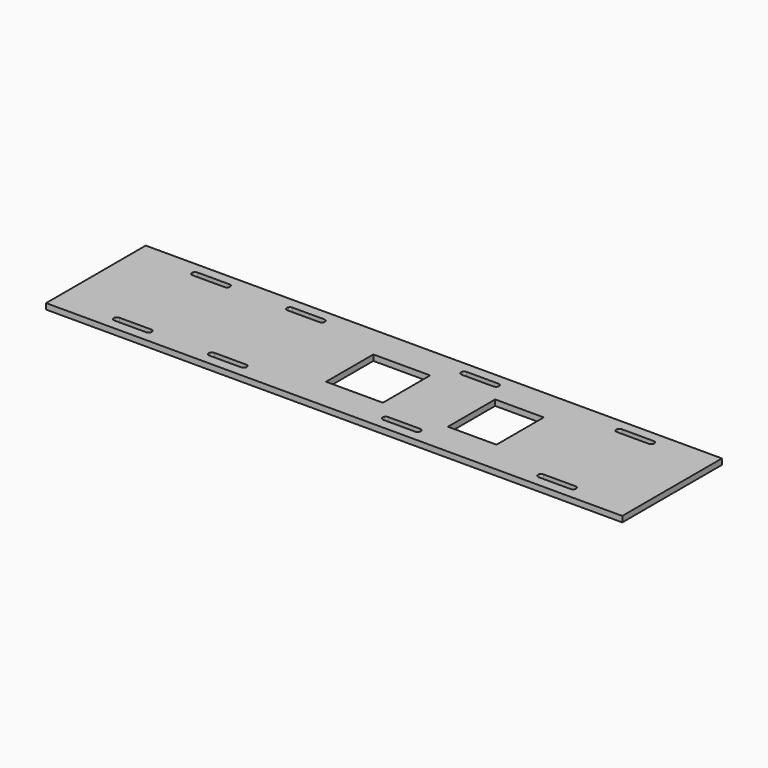
from build123d import *

# Parameters (mm, degrees)
F0_W     = 240.88725
F0_H     = 52.080583
F0_W_2   = 23.749
F0_H_2   = 24.712083
F0_W_3   = 20.32
F1_DEPTH = 2.4


# Not quite as in the source:
# - ends of sketch curves that miss each other by under 0.0002 mm in the source are joined


with BuildPart() as f1:
    # F0 (on Top) → F1 (new body)
    with BuildSketch(Plane.XY):
        with Locations((0, 5e-07)):
            Rectangle(F0_W, F0_H)
        with BuildLine():
            add(Edge.make_bspline(
                [(-95.3406640139, -19.1717048442), (-95.7930787698, -19.173702026), (-96.2109496029, -19.415645799), (-96.438113, -19.80762)],
                knots=[0.0087343308, 0.0087343308, 0.0087343308, 0.0087343308, 1, 1, 1, 1], degree=3))
            Line((-95.3406640139, -19.1717048442), (-95.328697, -19.171708))
            Line((-95.328697, -19.171708), (-82.016247, -19.171708))
            add(Edge.make_bspline(
                [(-80.906831, -19.807617), (-81.135996, -19.412192), (-81.559244, -19.16956), (-82.016247, -19.171708)],
                knots=[0, 0, 0, 0, 1, 1, 1, 1], degree=3))
            add(Edge.make_bspline(
                [(-80.906831, -21.086383), (-80.677667, -20.690913), (-80.677667, -20.203086), (-80.906831, -19.807617)],
                knots=[0, 0, 0, 0, 1, 1, 1, 1], degree=3))
            add(Edge.make_bspline(
                [(-82.0155410145, -21.7222942934), (-81.5588081414, -21.7242989555), (-81.1358779896, -21.4816033731), (-80.906831, -21.086383)],
                knots=[0.0005149583, 0.0005149583, 0.0005149583, 0.0005149583, 1, 1, 1, 1], degree=3))
            add(Edge.make_bspline(
                [(-82.016247, -21.722291), (-82.0160116625, -21.7222921628), (-82.015776334, -21.7222932606), (-82.0155410145, -21.7222942934)],
                knots=[0, 0, 0, 0, 0.0005149583, 0.0005149583, 0.0005149583, 0.0005149583], degree=3))
            Line((-82.016247, -21.722291), (-95.328697, -21.722291))
            add(Edge.make_bspline(
                [(-95.339958014, -21.7222944098), (-95.336206682, -21.7223097734), (-95.3324529811, -21.7223086538), (-95.328697, -21.722291)],
                knots=[0.991781277, 0.991781277, 0.991781277, 0.991781277, 1, 1, 1, 1], degree=3))
            add(Edge.make_bspline(
                [(-96.438113, -21.086383), (-96.2108314436, -21.4785571197), (-95.7926440063, -21.7204404289), (-95.339958014, -21.7222944098)],
                knots=[0, 0, 0, 0, 0.991781277, 0.991781277, 0.991781277, 0.991781277], degree=3))
            add(Edge.make_bspline(
                [(-96.438113, -19.80762), (-96.667277, -20.203086), (-96.667277, -20.690913), (-96.438113, -21.086383)],
                knots=[0, 0, 0, 0, 1, 1, 1, 1], degree=3))
        make_face(mode=Mode.SUBTRACT)
        with BuildLine():
            add(Edge.make_bspline(
                [(-55.6425800139, -19.1717048399), (-56.0949941873, -19.1737016787), (-56.5128664399, -19.4156455176), (-56.74003, -19.80762)],
                knots=[0.0087336193, 0.0087336193, 0.0087336193, 0.0087336193, 1, 1, 1, 1], degree=3))
            Line((-55.6425800139, -19.1717048399), (-55.630614, -19.171708))
            Line((-55.630614, -19.171708), (-42.30758, -19.171708))
            add(Edge.make_bspline(
                [(-41.198165, -19.807617), (-41.427329, -19.412192), (-41.850578, -19.16956), (-42.30758, -19.171708)],
                knots=[0, 0, 0, 0, 1, 1, 1, 1], degree=3))
            add(Edge.make_bspline(
                [(-41.198165, -21.086383), (-40.969, -20.690913), (-40.969, -20.203086), (-41.198165, -19.807617)],
                knots=[0, 0, 0, 0, 1, 1, 1, 1], degree=3))
            add(Edge.make_bspline(
                [(-42.3068750144, -21.722294289), (-41.8501427567, -21.7242993092), (-41.427211157, -21.4816036611), (-41.198165, -21.086383)],
                knots=[0.00051423, 0.00051423, 0.00051423, 0.00051423, 1, 1, 1, 1], degree=3))
            add(Edge.make_bspline(
                [(-42.30758, -21.722291), (-42.3073449959, -21.7222921611), (-42.3071100007, -21.7222932575), (-42.3068750144, -21.722294289)],
                knots=[0, 0, 0, 0, 0.00051423, 0.00051423, 0.00051423, 0.00051423], degree=3))
            Line((-42.30758, -21.722291), (-55.630614, -21.722291))
            add(Edge.make_bspline(
                [(-55.641875014, -21.7222944097), (-55.6381236819, -21.7223097734), (-55.6343699809, -21.7223086539), (-55.630614, -21.722291)],
                knots=[0.9917812593, 0.9917812593, 0.9917812593, 0.9917812593, 1, 1, 1, 1], degree=3))
            add(Edge.make_bspline(
                [(-56.74003, -21.086383), (-56.5127484477, -21.4785571127), (-56.0945600376, -21.7204404203), (-55.641875014, -21.7222944097)],
                knots=[0, 0, 0, 0, 0.9917812593, 0.9917812593, 0.9917812593, 0.9917812593], degree=3))
            add(Edge.make_bspline(
                [(-56.74003, -19.80762), (-56.969194, -20.203086), (-56.969194, -20.690913), (-56.74003, -21.086383)],
                knots=[0, 0, 0, 0, 1, 1, 1, 1], degree=3))
        make_face(mode=Mode.SUBTRACT)
        with BuildLine():
            add(Edge.make_bspline(
                [(17.0966689861, -19.1717048443), (16.644255197, -19.1737020352), (16.2263833928, -19.4156458064), (15.99922, -19.80762)],
                knots=[0.0087343496, 0.0087343496, 0.0087343496, 0.0087343496, 1, 1, 1, 1], degree=3))
            Line((17.0966689861, -19.1717048443), (17.108636, -19.171708))
            Line((17.108636, -19.171708), (30.421086, -19.171708))
            add(Edge.make_bspline(
                [(31.530502, -19.807617), (31.301338, -19.412192), (30.878089, -19.16956), (30.421086, -19.171708)],
                knots=[0, 0, 0, 0, 1, 1, 1, 1], degree=3))
            add(Edge.make_bspline(
                [(31.530502, -21.086383), (31.759666, -20.690913), (31.759666, -20.203086), (31.530502, -19.807617)],
                knots=[0, 0, 0, 0, 1, 1, 1, 1], degree=3))
            add(Edge.make_bspline(
                [(30.4217919855, -21.7222942934), (30.8785248597, -21.7242989555), (31.3014560099, -21.4816033731), (31.530502, -21.086383)],
                knots=[0.0005149583, 0.0005149583, 0.0005149583, 0.0005149583, 1, 1, 1, 1], degree=3))
            add(Edge.make_bspline(
                [(30.421086, -21.722291), (30.4213213375, -21.7222921628), (30.421556666, -21.7222932606), (30.4217919855, -21.7222942934)],
                knots=[0, 0, 0, 0, 0.0005149583, 0.0005149583, 0.0005149583, 0.0005149583], degree=3))
            Line((30.421086, -21.722291), (17.108636, -21.722291))
            add(Edge.make_bspline(
                [(17.097374986, -21.7222944097), (17.1011263181, -21.7223097734), (17.1048800191, -21.7223086539), (17.108636, -21.722291)],
                knots=[0.9917812593, 0.9917812593, 0.9917812593, 0.9917812593, 1, 1, 1, 1], degree=3))
            add(Edge.make_bspline(
                [(15.99922, -21.086383), (16.2265015523, -21.4785571127), (16.6446899624, -21.7204404203), (17.097374986, -21.7222944097)],
                knots=[0, 0, 0, 0, 0.9917812593, 0.9917812593, 0.9917812593, 0.9917812593], degree=3))
            add(Edge.make_bspline(
                [(15.99922, -19.80762), (15.770056, -20.203086), (15.770056, -20.690913), (15.99922, -21.086383)],
                knots=[0, 0, 0, 0, 1, 1, 1, 1], degree=3))
        make_face(mode=Mode.SUBTRACT)
        with BuildLine():
            add(Edge.make_bspline(
                [(82.0148359861, -19.1717048442), (81.5624212302, -19.173702026), (81.1445503971, -19.415645799), (80.917387, -19.80762)],
                knots=[0.0087343308, 0.0087343308, 0.0087343308, 0.0087343308, 1, 1, 1, 1], degree=3))
            Line((82.0148359861, -19.1717048442), (82.026803, -19.171708))
            Line((82.026803, -19.171708), (95.349836, -19.171708))
            add(Edge.make_bspline(
                [(96.459252, -19.807617), (96.230088, -19.412192), (95.806839, -19.16956), (95.349836, -19.171708)],
                knots=[0, 0, 0, 0, 1, 1, 1, 1], degree=3))
            add(Edge.make_bspline(
                [(96.459252, -21.086383), (96.688416, -20.690913), (96.688416, -20.203086), (96.459252, -19.807617)],
                knots=[0, 0, 0, 0, 1, 1, 1, 1], degree=3))
            add(Edge.make_bspline(
                [(95.3505419855, -21.7222942934), (95.8072748597, -21.7242989555), (96.2302060099, -21.4816033731), (96.459252, -21.086383)],
                knots=[0.0005149583, 0.0005149583, 0.0005149583, 0.0005149583, 1, 1, 1, 1], degree=3))
            add(Edge.make_bspline(
                [(95.349836, -21.722291), (95.3500713375, -21.7222921628), (95.350306666, -21.7222932606), (95.3505419855, -21.7222942934)],
                knots=[0, 0, 0, 0, 0.0005149583, 0.0005149583, 0.0005149583, 0.0005149583], degree=3))
            Line((95.349836, -21.722291), (82.026803, -21.722291))
            add(Edge.make_bspline(
                [(82.015541986, -21.7222944098), (82.019293318, -21.7223097734), (82.0230470189, -21.7223086538), (82.026803, -21.722291)],
                knots=[0.991781277, 0.991781277, 0.991781277, 0.991781277, 1, 1, 1, 1], degree=3))
            add(Edge.make_bspline(
                [(80.917387, -21.086383), (81.1446685564, -21.4785571197), (81.5628559937, -21.7204404289), (82.015541986, -21.7222944098)],
                knots=[0, 0, 0, 0, 0.991781277, 0.991781277, 0.991781277, 0.991781277], degree=3))
            add(Edge.make_bspline(
                [(80.917387, -19.80762), (80.688223, -20.203086), (80.688223, -20.690913), (80.917387, -21.086383)],
                knots=[0, 0, 0, 0, 1, 1, 1, 1], degree=3))
        make_face(mode=Mode.SUBTRACT)
        with Locations((-2.460625, 5e-07)):
            Rectangle(F0_W_2, F0_H_2, mode=Mode.SUBTRACT)
        with BuildLine():
            Line((-95.328697, 19.182292), (-95.339958, 19.182292))
            add(Edge.make_bspline(
                [(-96.438113, 19.818201), (-96.2108314436, 19.4260258885), (-95.7926440063, 19.1841425712), (-95.339958, 19.182292)],
                knots=[0, 0, 0, 0, 0.991781277, 0.991781277, 0.991781277, 0.991781277], degree=3))
            add(Edge.make_bspline(
                [(-96.438113, 21.096964), (-96.667277, 20.701497), (-96.667277, 20.21367), (-96.438113, 19.818201)],
                knots=[0, 0, 0, 0, 1, 1, 1, 1], degree=3))
            add(Edge.make_bspline(
                [(-95.3406640139, 21.7328781558), (-95.7930787698, 21.730880974), (-96.2109496029, 21.4889372098), (-96.438113, 21.096964)],
                knots=[0.0087343308, 0.0087343308, 0.0087343308, 0.0087343308, 1, 1, 1, 1], degree=3))
            add(Edge.make_bspline(
                [(-95.328697, 21.732875), (-95.3326886154, 21.7328947221), (-95.3366776556, 21.7328957535), (-95.3406640139, 21.7328781558)],
                knots=[0, 0, 0, 0, 0.0087343308, 0.0087343308, 0.0087343308, 0.0087343308], degree=3))
            Line((-95.328697, 21.732875), (-82.016247, 21.732875))
            add(Edge.make_bspline(
                [(-80.906831, 21.096967), (-81.135996, 21.492391), (-81.559244, 21.735023), (-82.016247, 21.732875)],
                knots=[0, 0, 0, 0, 1, 1, 1, 1], degree=3))
            add(Edge.make_bspline(
                [(-80.906831, 19.818201), (-80.677667, 20.21367), (-80.677667, 20.701497), (-80.906831, 21.096967)],
                knots=[0, 0, 0, 0, 1, 1, 1, 1], degree=3))
            add(Edge.make_bspline(
                [(-82.0155410145, 19.1822887066), (-81.5588081414, 19.1802840445), (-81.1358779896, 19.4229796274), (-80.906831, 19.818201)],
                knots=[0.0005149583, 0.0005149583, 0.0005149583, 0.0005149583, 1, 1, 1, 1], degree=3))
            Line((-82.0155410145, 19.1822887066), (-82.016247, 19.182292))
            Line((-82.016247, 19.182292), (-95.328697, 19.182292))
        make_face(mode=Mode.SUBTRACT)
        with BuildLine():
            Line((-55.630614, 19.182292), (-55.641875, 19.182292))
            add(Edge.make_bspline(
                [(-56.74003, 19.818201), (-56.5127484477, 19.4260258955), (-56.0945600376, 19.1841425798), (-55.641875, 19.182292)],
                knots=[0, 0, 0, 0, 0.9917812593, 0.9917812593, 0.9917812593, 0.9917812593], degree=3))
            add(Edge.make_bspline(
                [(-56.74003, 21.096964), (-56.969194, 20.701497), (-56.969194, 20.21367), (-56.74003, 19.818201)],
                knots=[0, 0, 0, 0, 1, 1, 1, 1], degree=3))
            add(Edge.make_bspline(
                [(-55.6425800139, 21.7328781601), (-56.0949941873, 21.7308813214), (-56.5128664399, 21.4889374911), (-56.74003, 21.096964)],
                knots=[0.0087336193, 0.0087336193, 0.0087336193, 0.0087336193, 1, 1, 1, 1], degree=3))
            add(Edge.make_bspline(
                [(-55.630614, 21.732875), (-55.6346052815, 21.7328947205), (-55.6385939884, 21.7328957534), (-55.6425800139, 21.7328781601)],
                knots=[0, 0, 0, 0, 0.0087336193, 0.0087336193, 0.0087336193, 0.0087336193], degree=3))
            Line((-55.630614, 21.732875), (-42.30758, 21.732875))
            add(Edge.make_bspline(
                [(-41.198165, 21.096967), (-41.427329, 21.492391), (-41.850578, 21.735023), (-42.30758, 21.732875)],
                knots=[0, 0, 0, 0, 1, 1, 1, 1], degree=3))
            add(Edge.make_bspline(
                [(-41.198165, 19.818201), (-40.969, 20.21367), (-40.969, 20.701497), (-41.198165, 21.096967)],
                knots=[0, 0, 0, 0, 1, 1, 1, 1], degree=3))
            add(Edge.make_bspline(
                [(-42.3068750144, 19.182288711), (-41.8501427567, 19.1802836908), (-41.427211157, 19.4229793394), (-41.198165, 19.818201)],
                knots=[0.00051423, 0.00051423, 0.00051423, 0.00051423, 1, 1, 1, 1], degree=3))
            Line((-42.3068750144, 19.182288711), (-42.30758, 19.182292))
            Line((-42.30758, 19.182292), (-55.630614, 19.182292))
        make_face(mode=Mode.SUBTRACT)
        with Locations((46.751875, 5e-07)):
            Rectangle(F0_W_3, F0_H_2, mode=Mode.SUBTRACT)
        with BuildLine():
            Line((17.108636, 19.182292), (17.097375, 19.182292))
            add(Edge.make_bspline(
                [(15.99922, 19.818201), (16.2265015523, 19.4260258955), (16.6446899624, 19.1841425798), (17.097375, 19.182292)],
                knots=[0, 0, 0, 0, 0.9917812593, 0.9917812593, 0.9917812593, 0.9917812593], degree=3))
            add(Edge.make_bspline(
                [(15.99922, 21.096964), (15.770056, 20.701497), (15.770056, 20.21367), (15.99922, 19.818201)],
                knots=[0, 0, 0, 0, 1, 1, 1, 1], degree=3))
            add(Edge.make_bspline(
                [(17.0966689861, 21.7328781557), (16.644255197, 21.7308809649), (16.2263833928, 21.4889372023), (15.99922, 21.096964)],
                knots=[0.0087343496, 0.0087343496, 0.0087343496, 0.0087343496, 1, 1, 1, 1], degree=3))
            add(Edge.make_bspline(
                [(17.108636, 21.732875), (17.1046443848, 21.7328947222), (17.1006553445, 21.7328957536), (17.0966689861, 21.7328781557)],
                knots=[0, 0, 0, 0, 0.0087343496, 0.0087343496, 0.0087343496, 0.0087343496], degree=3))
            Line((17.108636, 21.732875), (30.421086, 21.732875))
            add(Edge.make_bspline(
                [(31.530502, 21.096967), (31.301338, 21.492391), (30.878089, 21.735023), (30.421086, 21.732875)],
                knots=[0, 0, 0, 0, 1, 1, 1, 1], degree=3))
            add(Edge.make_bspline(
                [(31.530502, 19.818201), (31.759666, 20.21367), (31.759666, 20.701497), (31.530502, 21.096967)],
                knots=[0, 0, 0, 0, 1, 1, 1, 1], degree=3))
            add(Edge.make_bspline(
                [(30.4217919855, 19.1822887066), (30.8785248597, 19.1802840445), (31.3014560099, 19.4229796274), (31.530502, 19.818201)],
                knots=[0.0005149583, 0.0005149583, 0.0005149583, 0.0005149583, 1, 1, 1, 1], degree=3))
            Line((30.4217919855, 19.1822887066), (30.421086, 19.182292))
            Line((30.421086, 19.182292), (17.108636, 19.182292))
        make_face(mode=Mode.SUBTRACT)
        with BuildLine():
            Line((82.026803, 19.182292), (82.015542, 19.182292))
            add(Edge.make_bspline(
                [(80.917387, 19.818201), (81.1446685564, 19.4260258885), (81.5628559937, 19.1841425712), (82.015542, 19.182292)],
                knots=[0, 0, 0, 0, 0.991781277, 0.991781277, 0.991781277, 0.991781277], degree=3))
            add(Edge.make_bspline(
                [(80.917387, 21.096964), (80.688223, 20.701497), (80.688223, 20.21367), (80.917387, 19.818201)],
                knots=[0, 0, 0, 0, 1, 1, 1, 1], degree=3))
            add(Edge.make_bspline(
                [(82.0148359861, 21.7328781558), (81.5624212302, 21.730880974), (81.1445503971, 21.4889372098), (80.917387, 21.096964)],
                knots=[0.0087343308, 0.0087343308, 0.0087343308, 0.0087343308, 1, 1, 1, 1], degree=3))
            add(Edge.make_bspline(
                [(82.026803, 21.732875), (82.0228113846, 21.7328947221), (82.0188223444, 21.7328957535), (82.0148359861, 21.7328781558)],
                knots=[0, 0, 0, 0, 0.0087343308, 0.0087343308, 0.0087343308, 0.0087343308], degree=3))
            Line((82.026803, 21.732875), (95.349836, 21.732875))
            add(Edge.make_bspline(
                [(96.459252, 21.096967), (96.230088, 21.492391), (95.806839, 21.735023), (95.349836, 21.732875)],
                knots=[0, 0, 0, 0, 1, 1, 1, 1], degree=3))
            add(Edge.make_bspline(
                [(96.459252, 19.818201), (96.688416, 20.21367), (96.688416, 20.701497), (96.459252, 21.096967)],
                knots=[0, 0, 0, 0, 1, 1, 1, 1], degree=3))
            add(Edge.make_bspline(
                [(95.3505419855, 19.1822887066), (95.8072748597, 19.1802840445), (96.2302060099, 19.4229796274), (96.459252, 19.818201)],
                knots=[0.0005149583, 0.0005149583, 0.0005149583, 0.0005149583, 1, 1, 1, 1], degree=3))
            Line((95.3505419855, 19.1822887066), (95.349836, 19.182292))
            Line((95.349836, 19.182292), (82.026803, 19.182292))
        make_face(mode=Mode.SUBTRACT)
    extrude(amount=F1_DEPTH)


solid = f1.part
